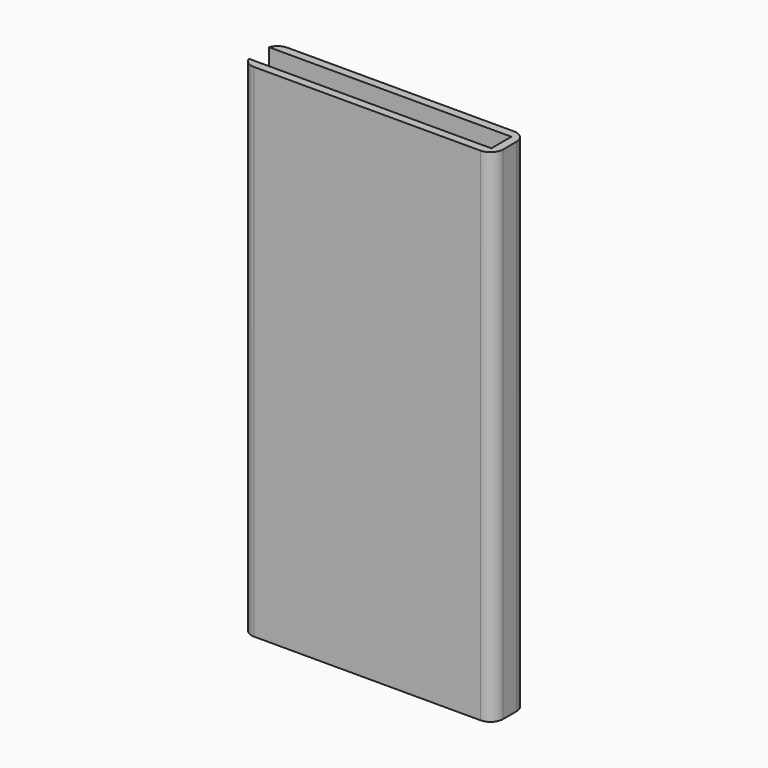
from build123d import *

# Parameters (mm, degrees)
F1_DEPTH    = 76.2
F2_T1_DEPTH = 85.725
F2_T3_DEPTH = 85.1802561211


# Not quite as in the source:
# - a fillet or chamfer that OpenCascade refuses, or shapes differently, is made with other operations: its cross-section is extruded or revolved along the edge and cut away or added


with BuildPart() as f1:
    # F0 (on Top) → F1 (new body)
    with BuildSketch(Plane.XY):
        Polygon((-19.05, -3.175), (19.05, -3.175), (19.05, 3.175), (-19.05, 3.175), (-19.05, 1.905), (17.78, 1.905), (17.78, -1.905), (-19.05, -1.905), align=None)
    extrude(amount=F1_DEPTH)

    # F2: fillet of radius 1.905 on 4 edges, made by hand

    # F2_s2 → F2_t1 (cut)
    with BuildSketch(Plane.XY.offset(-4.7625)):
        with BuildLine():
            ThreePointArc((19.05, 1.27), (18.4920384182, 2.6170384182), (17.145, 3.175))
            Line((17.145, 3.175), (19.05, 3.175))
            Line((19.05, 3.175), (19.05, 1.27))
        make_face()
        with BuildLine():
            ThreePointArc((17.145, -3.175), (18.4920384182, -2.6170384182), (19.05, -1.27))
            Line((19.05, -1.27), (19.05, -3.175))
            Line((19.05, -3.175), (17.145, -3.175))
        make_face()
    extrude(amount=F2_T1_DEPTH, mode=Mode.SUBTRACT)

    # F2_s4 → F2_t3 (cut)
    with BuildSketch(Plane.XY.offset(-4.4901280605)):
        with BuildLine():
            ThreePointArc((-19.05, -1.905), (-18.3538010386, -2.8254259867), (-17.2539487758, -3.175))
            Line((-17.2539487758, -3.175), (-19.05, -3.175))
            Line((-19.05, -3.175), (-19.05, -1.905))
        make_face()
        with BuildLine():
            ThreePointArc((-17.2539487758, 3.175), (-18.3538010386, 2.8254259867), (-19.05, 1.905))
            Line((-19.05, 1.905), (-19.05, 3.175))
            Line((-19.05, 3.175), (-17.2539487758, 3.175))
        make_face()
    extrude(amount=F2_T3_DEPTH, mode=Mode.SUBTRACT)


solid = f1.part
